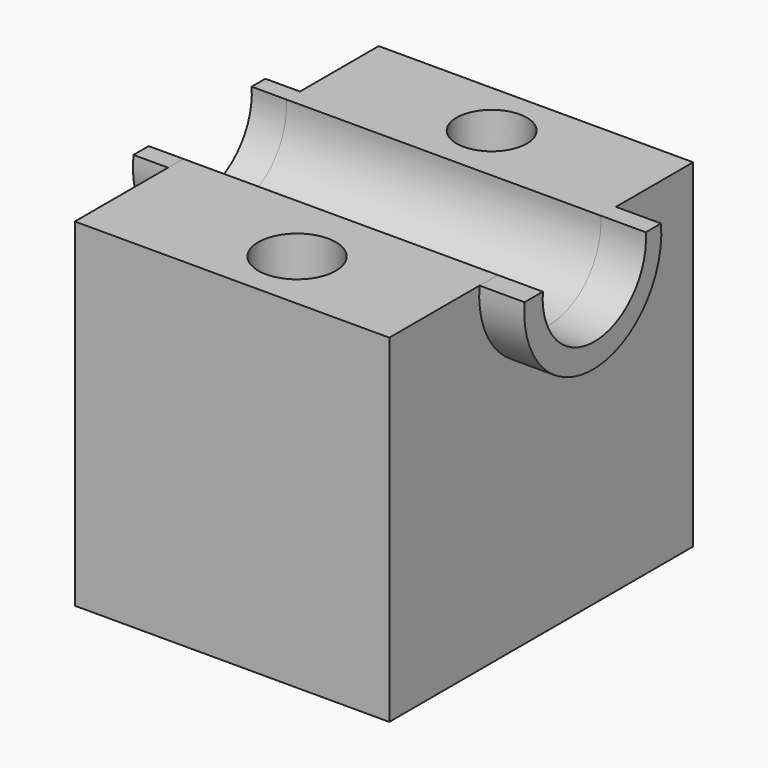
from build123d import *
from build123d import SkipClean  # not in build123d's __all__

# Parameters (mm, degrees)
F0_W     = 99.2605239153
F0_H     = 106.7802645266
F1_DEPTH = 59.944
F3_DEPTH = 99.2615239153
F5_DEPTH = 14.224
F7_DEPTH = 10.922
F8_R     = 11.0925650774
F8_R_2   = 12.2440148534
F9_DEPTH = 106.7812645266


# Not quite as in the source:
# - after a boolean that leaves OpenCascade's solid faulty, fix() repairs it


with BuildPart() as f1:
    # F0 (on Front) → F1 (new body, symmetric)
    with BuildSketch(Plane.XZ):
        with Locations((5.4142102599, -9.7756590694)):
            Rectangle(F0_W, F0_H)
    extrude(amount=F1_DEPTH, both=True)

    # F2 (on face) → F3 (cut, through all)
    with BuildSketch(Plane.YZ.offset(55.0444722176)):
        with BuildLine():
            Line((23.4615784138, 43.6144731939), (-17.1450003982, 43.6144731939))
            ThreePointArc((-17.1450003982, 43.6144731939), (3.1582890078, 21.4579654327), (23.4615784138, 43.6144731939))
        make_face()
    extrude(amount=-F3_DEPTH, mode=Mode.SUBTRACT)

    # F4 (on face) → F5 (join)
    with BuildSketch(Plane.YZ.offset(55.0444722176)):
        with BuildLine():
            Line((-17.1450003982, 43.6144731939), (-24.3639480323, 43.6144731939))
            ThreePointArc((-24.3639480323, 43.6144731939), (2.5567095727, 13.9394518293), (29.4773671776, 43.6144731939))
            Line((29.4773671776, 43.6144731939), (23.4615784138, 43.6144731939))
            ThreePointArc((23.4615784138, 43.6144731939), (3.1582890078, 21.4579654327), (-17.1450003982, 43.6144731939))
        make_face()
    with SkipClean():  # cleaning this boolean's faces spoils the solid; the shape is the same uncleaned
        extrude(amount=F5_DEPTH)

    # F6 (on face) → F7 (join)
    with BuildSketch(Plane(origin=(-44.2160516977, 0, 0), x_dir=(0, -1, 0), z_dir=(-1, 0, 0))):
        with BuildLine():
            Line((-23.4615784138, 43.6144731939), (-28.8757905364, 43.6144731939))
            ThreePointArc((-28.8757905364, 43.6144731939), (-2.8575006872, 14.036395677), (23.1607891619, 43.6144731939))
            Line((23.1607891619, 43.6144731939), (17.1450003982, 43.6144731939))
            ThreePointArc((17.1450003982, 43.6144731939), (-3.1582890078, 21.4579654327), (-23.4615784138, 43.6144731939))
        make_face()
    extrude(amount=F7_DEPTH)

    add(f1.part.fix(), mode=Mode.REPLACE)

    # F8 (on face) → F9 (cut, through all)
    with BuildSketch(Plane.XY.offset(43.6144731939)):
        with Locations((5.7150018401, 42.1105287969)):
            Circle(F8_R)
        with Locations((10.2268429473, -40.3057895601)):
            Circle(F8_R_2)
    extrude(amount=-F9_DEPTH, mode=Mode.SUBTRACT)


solid = f1.part
